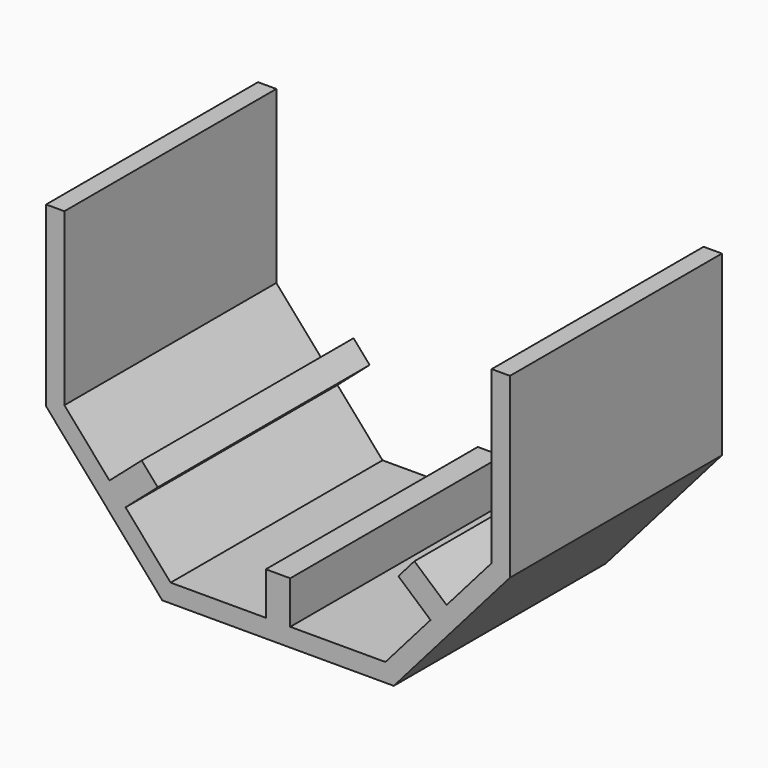
from build123d import *

# Parameters (mm, degrees)
F1_DEPTH = 217


# Not quite as in the source:
# - ends of sketch curves that miss each other by under 0.0002 mm in the source are joined


with BuildPart() as f1:
    # F0 (on Front) → F1 (new body)
    with BuildSketch(Plane.XZ):
        Polygon((-175, 127.260191), (-190, 127.260191), (-190, -18.260191), (-94.798649, -127.260191), (0, -127.260191), (94.798648, -127.260191), (190, -18.260191), (190, 127.260191), (175, 127.260191), (175, -12.631891), (138.0702256785, -54.9143307192), (111.7092396785, -31.8904637192), (98.552745, -46.953885), (124.9137303215, -69.9777512808), (87.983956, -112.260191), (10, -112.260191), (10, -77.260191), (-10, -77.260191), (-10, -112.260191), (-87.983957, -112.260191), (-124.9137310807, -69.9777510705), (-98.5527450807, -46.9538850705), (-111.70924, -31.890464), (-138.0702259193, -54.9143309295), (-175, -12.631891), align=None)
    extrude(amount=F1_DEPTH)


solid = f1.part
